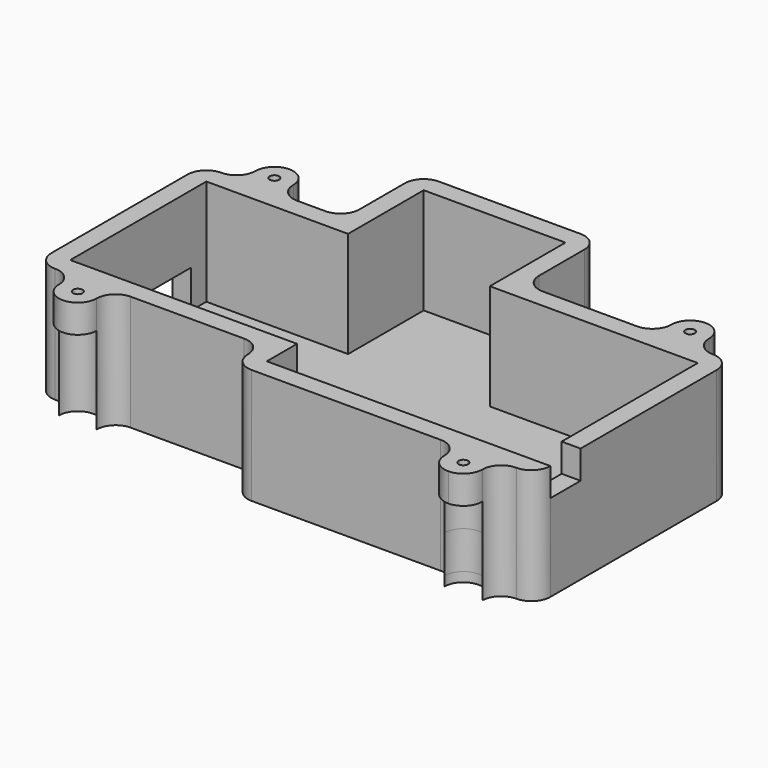
from build123d import *

# Parameters (mm, degrees)
F1_W      = 5
F1_H      = 10
F1_H_2    = 35
F2_DEPTH  = 2.5
F3_DEPTH  = 28
F5_D      = 2.5
F6_DEPTH  = 20.5
F7_DEPTH  = 18
F8_DEPTH  = 10
F9_R      = 1.25
F10_DEPTH = 23


with BuildPart() as f2:
    # F1 (on Top) → F2 (new body)
    with BuildSketch(Plane.XY):
        Polygon((0, 0), (70, 0), (70, 10), (70, 55), (15, 55), (15, 80), (-22.5, 80), (-22.5, 55), (-60, 55), (-60, 50), (-60, 15), (-60, 10), (0, 10), align=None)
        with BuildLine():
            Line((70, 10), (75, 10))
            Line((75, 10), (75, 55))
            ThreePointArc((75, 55), (73.5355339059, 58.5355339059), (70, 60))
            ThreePointArc((70, 60), (66.4644660941, 61.4644660941), (65, 65))
            ThreePointArc((65, 65), (60, 60), (55, 65))
            ThreePointArc((55, 65), (53.5355339059, 61.4644660941), (50, 60))
            Line((50, 60), (25, 60))
            ThreePointArc((25, 60), (21.4644660941, 61.4644660941), (20, 65))
            Line((20, 65), (20, 80))
            ThreePointArc((20, 80), (18.5355339059, 83.5355339059), (15, 85))
            Line((15, 85), (-22.5, 85))
            ThreePointArc((-22.5, 85), (-26.0355339059, 83.5355339059), (-27.5, 80))
            Line((-27.5, 80), (-27.5, 65))
            ThreePointArc((-27.5, 65), (-28.9644660941, 61.4644660941), (-32.5, 60))
            Line((-32.5, 60), (-40, 60))
            ThreePointArc((-40, 60), (-43.5355339059, 61.4644660941), (-45, 65))
            ThreePointArc((-45, 65), (-50, 60), (-55, 65))
            ThreePointArc((-55, 65), (-56.4644660941, 61.4644660941), (-60, 60))
            ThreePointArc((-60, 60), (-63.5355339059, 58.5355339059), (-65, 55))
            Line((-65, 55), (-65, 50))
            Line((-65, 50), (-60, 50))
            Line((-60, 50), (-60, 55))
            Line((-60, 55), (-22.5, 55))
            Line((-22.5, 55), (-22.5, 80))
            Line((-22.5, 80), (15, 80))
            Line((15, 80), (15, 55))
            Line((15, 55), (70, 55))
            Line((70, 55), (70, 10))
        make_face()
        with Locations((72.5, 5)):
            Rectangle(F1_W, F1_H)
        with BuildLine():
            ThreePointArc((-50, 70), (-53.5355339059, 68.5355339059), (-55, 65))
            ThreePointArc((-55, 65), (-50, 60), (-45, 65))
            ThreePointArc((-45, 65), (-46.4644660941, 68.5355339059), (-50, 70))
        make_face()
        with BuildLine():
            ThreePointArc((55, 65), (60, 60), (65, 65))
            ThreePointArc((65, 65), (63.5355339059, 68.5355339059), (60, 70))
            ThreePointArc((60, 70), (56.4644660941, 68.5355339059), (55, 65))
        make_face()
        with BuildLine():
            ThreePointArc((-45, 0), (-50, 5), (-55, 0))
            ThreePointArc((-55, 0), (-53.5355339059, -3.5355339059), (-50, -5))
            ThreePointArc((-50, -5), (-46.4644660941, -3.5355339059), (-45, 0))
        make_face()
        with Locations((-62.5, 32.5)):
            Rectangle(F1_W, F1_H_2)
        with BuildLine():
            ThreePointArc((70, -5), (73.5355339059, -3.5355339059), (75, 0))
            Line((75, 0), (70, 0))
            Line((70, 0), (0, 0))
            Line((0, 0), (0, 10))
            Line((0, 10), (-60, 10))
            Line((-60, 10), (-60, 15))
            Line((-60, 15), (-65, 15))
            Line((-65, 15), (-65, 10))
            ThreePointArc((-65, 10), (-63.5355339059, 6.4644660941), (-60, 5))
            ThreePointArc((-60, 5), (-56.4644660941, 3.5355339059), (-55, 0))
            ThreePointArc((-55, 0), (-50, 5), (-45, 0))
            ThreePointArc((-45, 0), (-43.5355339059, 3.5355339059), (-40, 5))
            Line((-40, 5), (-10, 5))
            ThreePointArc((-10, 5), (-6.4644660941, 3.5355339059), (-5, 0))
            ThreePointArc((-5, 0), (-3.5355339059, -3.5355339059), (0, -5))
            Line((0, -5), (50, -5))
            ThreePointArc((50, -5), (53.5355339059, -6.4644660941), (55, -10))
            ThreePointArc((55, -10), (56.4644660941, -6.4644660941), (60, -5))
            ThreePointArc((60, -5), (63.5355339059, -6.4644660941), (65, -10))
            ThreePointArc((65, -10), (66.4644660941, -6.4644660941), (70, -5))
        make_face()
    extrude(amount=-F2_DEPTH)

    # F1 (on Top) → F3 (join)
    with BuildSketch(Plane.XY):
        with BuildLine():
            ThreePointArc((70, -5), (73.5355339059, -3.5355339059), (75, 0))
            Line((75, 0), (70, 0))
            Line((70, 0), (0, 0))
            Line((0, 0), (0, 10))
            Line((0, 10), (-60, 10))
            Line((-60, 10), (-60, 15))
            Line((-60, 15), (-65, 15))
            Line((-65, 15), (-65, 10))
            ThreePointArc((-65, 10), (-63.5355339059, 6.4644660941), (-60, 5))
            ThreePointArc((-60, 5), (-56.4644660941, 3.5355339059), (-55, 0))
            ThreePointArc((-55, 0), (-50, 5), (-45, 0))
            ThreePointArc((-45, 0), (-43.5355339059, 3.5355339059), (-40, 5))
            Line((-40, 5), (-10, 5))
            ThreePointArc((-10, 5), (-6.4644660941, 3.5355339059), (-5, 0))
            ThreePointArc((-5, 0), (-3.5355339059, -3.5355339059), (0, -5))
            Line((0, -5), (50, -5))
            ThreePointArc((50, -5), (53.5355339059, -6.4644660941), (55, -10))
            ThreePointArc((55, -10), (56.4644660941, -6.4644660941), (60, -5))
            ThreePointArc((60, -5), (63.5355339059, -6.4644660941), (65, -10))
            ThreePointArc((65, -10), (66.4644660941, -6.4644660941), (70, -5))
        make_face()
        with BuildLine():
            Line((70, 10), (75, 10))
            Line((75, 10), (75, 55))
            ThreePointArc((75, 55), (73.5355339059, 58.5355339059), (70, 60))
            ThreePointArc((70, 60), (66.4644660941, 61.4644660941), (65, 65))
            ThreePointArc((65, 65), (60, 60), (55, 65))
            ThreePointArc((55, 65), (53.5355339059, 61.4644660941), (50, 60))
            Line((50, 60), (25, 60))
            ThreePointArc((25, 60), (21.4644660941, 61.4644660941), (20, 65))
            Line((20, 65), (20, 80))
            ThreePointArc((20, 80), (18.5355339059, 83.5355339059), (15, 85))
            Line((15, 85), (-22.5, 85))
            ThreePointArc((-22.5, 85), (-26.0355339059, 83.5355339059), (-27.5, 80))
            Line((-27.5, 80), (-27.5, 65))
            ThreePointArc((-27.5, 65), (-28.9644660941, 61.4644660941), (-32.5, 60))
            Line((-32.5, 60), (-40, 60))
            ThreePointArc((-40, 60), (-43.5355339059, 61.4644660941), (-45, 65))
            ThreePointArc((-45, 65), (-50, 60), (-55, 65))
            ThreePointArc((-55, 65), (-56.4644660941, 61.4644660941), (-60, 60))
            ThreePointArc((-60, 60), (-63.5355339059, 58.5355339059), (-65, 55))
            Line((-65, 55), (-65, 50))
            Line((-65, 50), (-60, 50))
            Line((-60, 50), (-60, 55))
            Line((-60, 55), (-22.5, 55))
            Line((-22.5, 55), (-22.5, 80))
            Line((-22.5, 80), (15, 80))
            Line((15, 80), (15, 55))
            Line((15, 55), (70, 55))
            Line((70, 55), (70, 10))
        make_face()
        with BuildLine():
            ThreePointArc((60, -15), (63.5355339059, -13.5355339059), (65, -10))
            ThreePointArc((65, -10), (63.5355339059, -6.4644660941), (60, -5))
            ThreePointArc((60, -5), (56.4644660941, -6.4644660941), (55, -10))
            ThreePointArc((55, -10), (56.4644660941, -13.5355339059), (60, -15))
        make_face()
        with BuildLine():
            ThreePointArc((55, 65), (60, 60), (65, 65))
            ThreePointArc((65, 65), (63.5355339059, 68.5355339059), (60, 70))
            ThreePointArc((60, 70), (56.4644660941, 68.5355339059), (55, 65))
        make_face()
        with Locations((-62.5, 32.5)):
            Rectangle(F1_W, F1_H_2)
        with BuildLine():
            ThreePointArc((-45, 0), (-50, 5), (-55, 0))
            ThreePointArc((-55, 0), (-53.5355339059, -3.5355339059), (-50, -5))
            ThreePointArc((-50, -5), (-46.4644660941, -3.5355339059), (-45, 0))
        make_face()
        with BuildLine():
            ThreePointArc((-50, 70), (-53.5355339059, 68.5355339059), (-55, 65))
            ThreePointArc((-55, 65), (-50, 60), (-45, 65))
            ThreePointArc((-45, 65), (-46.4644660941, 68.5355339059), (-50, 70))
        make_face()
    extrude(amount=F3_DEPTH)

    # F5 (through all)
    with Locations(Plane(origin=(0, 0, -2.5), x_dir=(1, 0, 0), z_dir=(0, 0, -1))):
        with Locations((-50, 0), (60, 10), (60, -65), (-50, -65)):
            Hole(F5_D / 2)

    # F1 (on Top) → F6 (join)
    with BuildSketch(Plane.XY):
        with Locations((72.5, 5)):
            Rectangle(F1_W, F1_H)
    extrude(amount=F6_DEPTH)

    # F0 (on Top) → F7 (join)
    with BuildSketch(Plane.XY):
        Polygon((15, 5), (15, 0), (35, 0), (35, 5), (35, 10), (15, 10), align=None)
        Polygon((35, 5), (35, 0), (70, 0), (70, 10), (35, 10), align=None)
    extrude(amount=F7_DEPTH)

    # F1 (on Top) → F8 (cut)
    with BuildSketch(Plane.XY):
        with BuildLine():
            ThreePointArc((60, -15), (63.5355339059, -13.5355339059), (65, -10))
            ThreePointArc((65, -10), (63.5355339059, -6.4644660941), (60, -5))
            ThreePointArc((60, -5), (56.4644660941, -6.4644660941), (55, -10))
            ThreePointArc((55, -10), (56.4644660941, -13.5355339059), (60, -15))
        make_face()
        with Locations((-62.5, 32.5)):
            Rectangle(F1_W, F1_H_2)
    extrude(amount=F8_DEPTH, mode=Mode.SUBTRACT)

    # F9 (on face) → F10 (cut)
    with BuildSketch(Plane(origin=(0, 0, -2.5), x_dir=(1, 0, 0), z_dir=(0, 0, -1))):
        with BuildLine():
            ThreePointArc((-55, 0), (-50, -5), (-45, 0))
            ThreePointArc((-45, 0), (-50, 5), (-55, 0))
        make_face()
        with Locations((-50, 0)):
            Circle(F9_R, mode=Mode.SUBTRACT)
        with BuildLine():
            ThreePointArc((-45, -65), (-50, -60), (-55, -65))
            ThreePointArc((-55, -65), (-50, -70), (-45, -65))
        make_face()
        with Locations((-50, -65)):
            Circle(F9_R, mode=Mode.SUBTRACT)
        with BuildLine():
            ThreePointArc((65, 10), (60, 15), (55, 10))
            ThreePointArc((55, 10), (60, 5), (65, 10))
        make_face()
        with BuildLine():
            ThreePointArc((55, -65), (60, -70), (65, -65))
            ThreePointArc((65, -65), (60, -60), (55, -65))
        make_face()
        with Locations((60, -65)):
            Circle(F9_R, mode=Mode.SUBTRACT)
    extrude(amount=-F10_DEPTH, mode=Mode.SUBTRACT)


solid = f2.part
